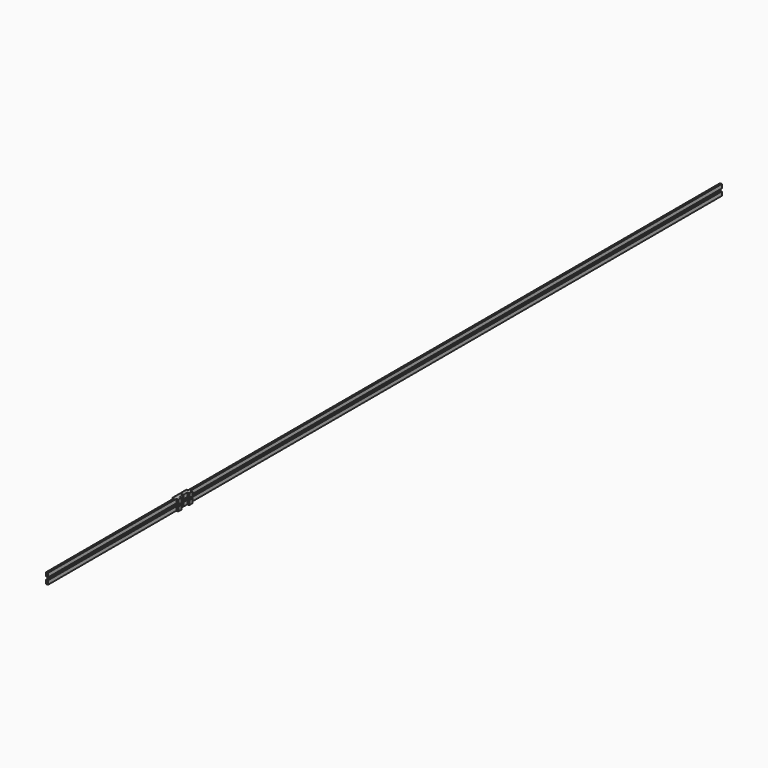
from build123d import *

# Parameters (mm, degrees)
F0_W      = 10
F0_H      = 20
F1_DEPTH  = 4302.45
F3_E6_W   = 25.4
F3_E6_H   = 9.525
F3_E5_W   = 25.4
F3_E5_H   = 9.525
F4_DEPTH  = 90
F7_DEPTH  = 10
F9_DEPTH  = 53.47
F10_R     = 5
F11_R     = 5
F12_DEPTH = 10
F14_DEPTH = 9.525


with BuildPart() as f1:
    # F0 (on Front) → F1 (new body)
    with BuildSketch(Plane.XZ):
        with Locations((-42.1546186507, 27.1410486561)):
            Rectangle(F0_W, F0_H)
        with Locations((-42.1546186507, -6.3289513439)):
            Rectangle(F0_W, F0_H)
    extrude(amount=F1_DEPTH)

    # F8 (on face) → F9 (cut, through all)
    with BuildSketch(Plane.XY.offset(37.1410486561)):
        Polygon((-47.1546186507, -3438.3331108093), (-47.1546186507, -3439.3331108093), (-37.1546186507, -3439.3331108093), (-37.1546186507, -3438.3331108093), (-37.1546186507, -3437.3331108093), (-47.1546186507, -3437.3331108093), align=None)
    extrude(amount=-F9_DEPTH, mode=Mode.SUBTRACT)


with BuildPart() as f4:
    # F3_E6 (on explicit) + F3_E5 (on explicit) → F4 (new body)
    with BuildSketch(Plane(origin=(-47.1546186507, -3483.3331108093, 10.4060486561), x_dir=(0, 0, -1), z_dir=(0, 1, 0))):
        with Locations((12.7, 4.7625)):
            Rectangle(F3_E6_W, F3_E6_H)
    with BuildSketch(Plane(origin=(-47.1546186507, -3483.3331108093, 35.8060486561), x_dir=(0, 0, -1), z_dir=(0, 1, 0))):
        with Locations((12.7, 4.7625)):
            Rectangle(F3_E5_W, F3_E5_H)
    extrude(amount=F4_DEPTH)

    # F13 (on face) + F5 (on face) → F14 (cut, through all)
    with BuildSketch(Plane(origin=(-56.6796186507, 0, 0), x_dir=(0, -1, 0), z_dir=(-1, 0, 0))):
        with BuildLine():
            Line((3408.3331108093, 15.4060486561), (3393.3331108093, 15.4060486561))
            Line((3393.3331108093, 15.4060486561), (3393.3331108093, 5.4060486561))
            Line((3393.3331108093, 5.4060486561), (3403.3331108093, 5.4060486561))
            Line((3403.3331108093, 5.4060486561), (3408.3331108093, 5.4060486561))
            ThreePointArc((3408.3331108093, 5.4060486561), (3413.3331108093, 10.4060486561), (3408.3331108093, 15.4060486561))
        make_face()
    with BuildSketch(Plane(origin=(-56.6796186507, 0, 0), x_dir=(0, -1, 0), z_dir=(-1, 0, 0))):
        with BuildLine():
            ThreePointArc((3468.3331108093, 15.4060486561), (3463.3331108093, 10.4060486561), (3468.3331108093, 5.4060486561))
            Line((3468.3331108093, 5.4060486561), (3473.3331108093, 5.4060486561))
            Line((3473.3331108093, 5.4060486561), (3483.3331108093, 5.4060486561))
            Line((3483.3331108093, 5.4060486561), (3483.3331108093, 15.4060486561))
            Line((3483.3331108093, 15.4060486561), (3468.3331108093, 15.4060486561))
        make_face()
    extrude(amount=-F14_DEPTH, mode=Mode.SUBTRACT)


with BuildPart() as f7:
    # F6 (on face) → F7 (new body)
    with BuildSketch(Plane.YZ.offset(-37.1546186507)):
        Polygon((-3483.3331108093, 37.1410486561), (-3483.3331108093, 35.8060486561), (-3483.3331108093, 15.4060486561), (-3483.3331108093, 5.4060486561), (-3483.3331108093, 3.6710486561), (-3463.3331108093, 3.6710486561), (-3463.3331108093, 37.1410486561), align=None)
        Polygon((-3463.3331108093, 3.6710486561), (-3483.3331108093, 3.6710486561), (-3483.3331108093, -14.9939513439), (-3483.3331108093, -16.3289513439), (-3463.3331108093, -16.3289513439), align=None)
        Polygon((-3393.3331108093, 37.1410486561), (-3413.3331108093, 37.1410486561), (-3413.3331108093, 3.6710486561), (-3393.3331108093, 3.6710486561), (-3393.3331108093, 5.4060486561), (-3393.3331108093, 15.4060486561), (-3393.3331108093, 35.8060486561), align=None)
        Polygon((-3393.3331108093, 3.6710486561), (-3413.3331108093, 3.6710486561), (-3413.3331108093, -16.3289513439), (-3393.3331108093, -16.3289513439), (-3393.3331108093, -14.9939513439), align=None)
    extrude(amount=F7_DEPTH)

    # F10 (on face) + F11 (on face) → F12 (cut)
    with BuildSketch(Plane.YZ.offset(-27.1546186507)):
        with Locations((-3473.3331108093, 10.4060486561)):
            Circle(F10_R)
    with BuildSketch(Plane.YZ.offset(-27.1546186507)):
        with Locations((-3403.3331108093, 10.4060486561)):
            Circle(F11_R)
    extrude(amount=-F12_DEPTH, mode=Mode.SUBTRACT)


solid = Compound([f1.part, f4.part, f7.part])
